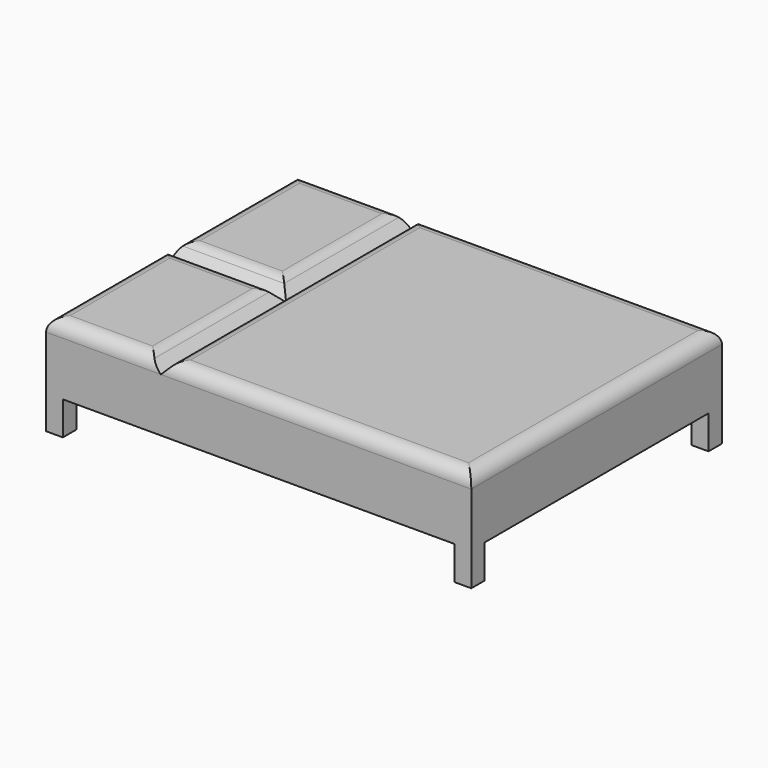
from build123d import *

# Parameters (mm, degrees)
F0_W     = 19
F0_H     = 14
F1_DEPTH = 3
F2_W     = 0.75
F2_H     = 0.75
F3_DEPTH = 1.5
F5_DEPTH = 14.001
F7_DEPTH = 5.127709538
F8_R     = 0.59999


# Not quite as in the source:
# - a fillet or chamfer is up to 0.001 mm smaller than in the source, because OpenCascade refuses the exact size


with BuildPart() as f1:
    # F0 (on Top) → F1 (new body)
    with BuildSketch(Plane.XY):
        Rectangle(F0_W, F0_H)
    extrude(amount=F1_DEPTH)

    # F2 (on face) → F3 (join)
    with BuildSketch(Plane(origin=(0, 0, 0), x_dir=(1, 0, 0), z_dir=(0, 0, -1))):
        with Locations((9.125, 6.625)):
            Rectangle(F2_W, F2_H)
        with Locations((-9.125, 6.625)):
            Rectangle(F2_W, F2_H)
        with Locations((-9.125, -6.625)):
            Rectangle(F2_W, F2_H)
        with Locations((9.125, -6.625)):
            Rectangle(F2_W, F2_H)
    extrude(amount=F3_DEPTH)

    # F4 (on face) → F5 (cut, through all)
    with BuildSketch(Plane.XZ.offset(7)):
        Polygon((-3.773290462, 3), (-4.973290462, 3), (-4.373290462, 2.4), align=None)
    extrude(amount=-F5_DEPTH, mode=Mode.SUBTRACT)

    # F6 (on face) → F7 (cut, through all)
    with BuildSketch(Plane(origin=(-9.5, 0, 0), x_dir=(0, -1, 0), z_dir=(-1, 0, 0))):
        Polygon((0.6, 3), (-0.6, 3), (0, 2.4), align=None)
    extrude(amount=-F7_DEPTH, mode=Mode.SUBTRACT)

    # F8 (radius 0.6 in the source; OpenCascade refuses exactly that, so slightly less here)
    f8_edges = [f1.edges().sort_by_distance(p)[0] for p in [
        (-3.77329, 0, 3),
        (-4.97329, 3.8, 3),
        (-4.97329, -3.8, 3),
        (-7.236645, -0.6, 3),
        (-7.236645, 0.6, 3),
        (2.863355, -7, 3),
        (-7.236645, -7, 3),
        (2.863355, 7, 3),
        (9.5, 0, 3),
        (-7.236645, 7, 3),
        (-9.5, 3.8, 3),
        (-9.5, -3.8, 3),
    ]]
    fillet(f8_edges, radius=F8_R)


solid = f1.part
